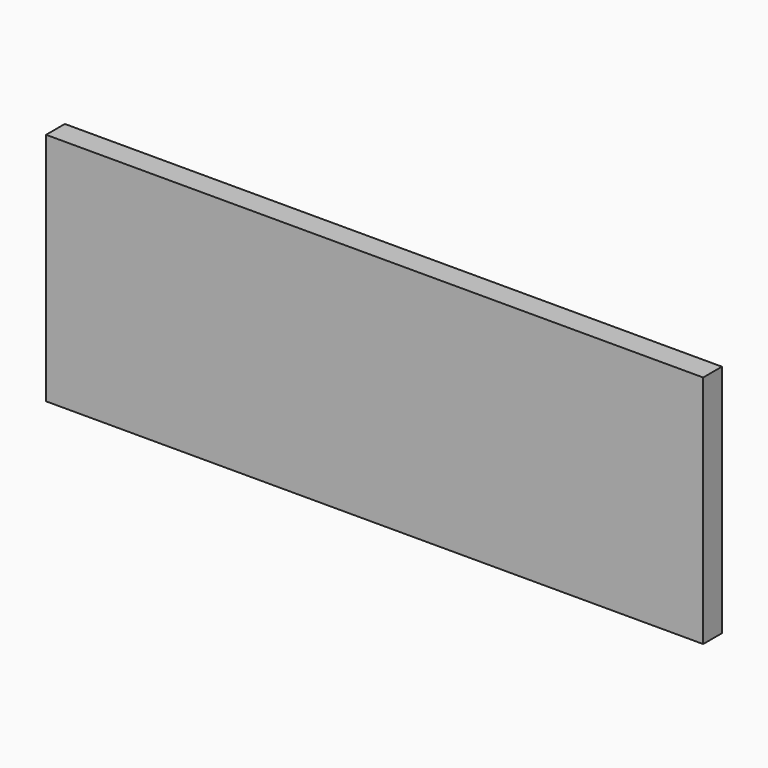
from build123d import *

# Parameters (mm, degrees)
F0_W     = 533.4
F0_H     = 190.5
F1_DEPTH = 19.05


# Not quite as in the source:
# - a feature names something its author has since deleted; it is built from what else it names


with BuildPart() as f1:
    # F0 (on Front) → F1 (new body)
    with BuildSketch(Plane.XZ):
        with Locations((266.7, 95.25)):
            Rectangle(F0_W, F0_H)
    extrude(amount=-F1_DEPTH)


solid = f1.part
